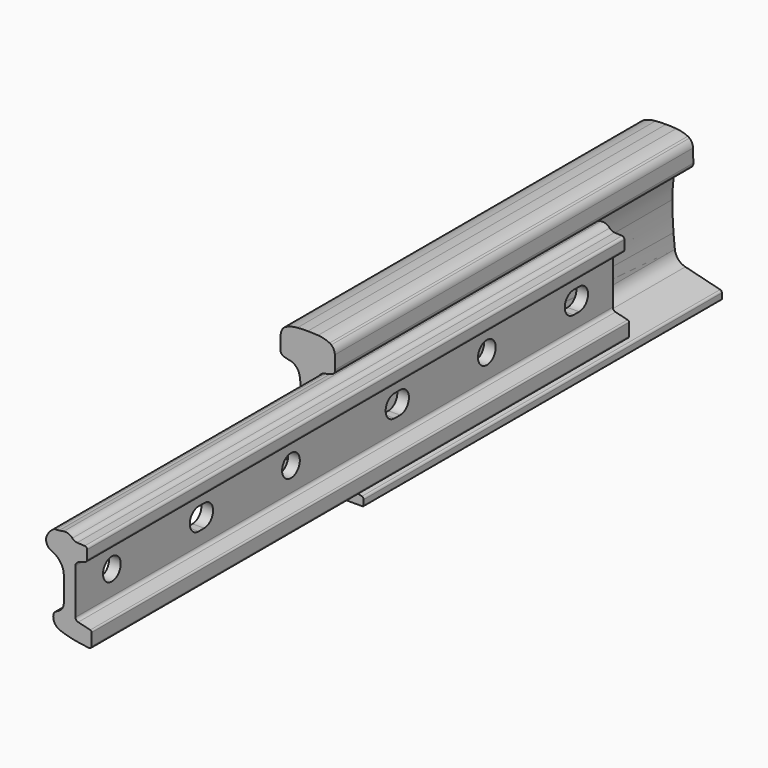
from build123d import *

# Parameters (mm, degrees)
F1_DEPTH  = 609.6
F4_DEPTH  = 609.6
F5_D      = 30.1625
F6_DEPTH  = 609.6
F7_D      = 30.1625
F10_DEPTH = 304.8
F3_R      = 15.08125
F11_DEPTH = 152.401
F12_DEPTH = 457.2
F13_DEPTH = 152.401


with BuildPart() as f1:
    # F0 (on Front) → F1 (new body)
    with BuildSketch(Plane.XZ):
        with BuildLine():
            Line((-74.6125, 0), (0, 0))
            Line((0, 0), (74.6125, 0))
            ThreePointArc((74.6125, 0), (75.7350320151, 0.4649679849), (76.2, 1.5875))
            Line((76.2, 1.5875), (76.2, 8.6375172708))
            ThreePointArc((76.2, 8.6375172708), (75.5275026433, 10.5915145891), (73.7948941606, 11.7177588168))
            Line((73.7948941606, 11.7177588168), (26.4239553104, 23.5579371467))
            ThreePointArc((26.4239553104, 23.5579371467), (16.7305028538, 29.4677613288), (12.1204139211, 39.842544335))
            ThreePointArc((12.1204139211, 39.842544335), (9.5792487577, 69.084794889), (8.73125, 98.425))
            ThreePointArc((8.73125, 98.425), (9.2653580474, 113.148322963), (10.8648744003, 127.7942458741))
            ThreePointArc((10.8648744003, 127.7942458741), (13.5406230824, 135.105519008), (18.917896304, 140.7357302429))
            ThreePointArc((18.917896304, 140.7357302429), (20.1528467839, 141.4316531197), (21.4918904061, 141.8968127872))
            Line((21.4918904061, 141.8968127872), (31.9637779941, 144.5142195666))
            ThreePointArc((31.9637779941, 144.5142195666), (35.8678959033, 147.0868819035), (37.30625, 151.5356868712))
            Line((37.30625, 151.5356868712), (36.8599990785, 169.3703104565))
            ThreePointArc((36.8599990785, 169.3703104565), (35.5405407375, 175.0194624076), (32.0838713197, 179.6783597682))
            ThreePointArc((32.0838713197, 179.6783597682), (30.9805783249, 180.5257181325), (29.765625, 181.2033316273))
            ThreePointArc((29.765625, 181.2033316273), (22.1130671826, 183.945655693), (14.0890625, 185.2484723667))
            ThreePointArc((14.0890625, 185.2484723667), (7.0487734776, 185.6152062911), (0, 185.7375))
            ThreePointArc((0, 185.7375), (-7.0487734776, 185.6152062911), (-14.0890625, 185.2484723667))
            ThreePointArc((-14.0890625, 185.2484723667), (-22.1130671826, 183.945655693), (-29.765625, 181.2033316273))
            ThreePointArc((-29.765625, 181.2033316273), (-30.9805783249, 180.5257181325), (-32.0838713197, 179.6783597682))
            ThreePointArc((-32.0838713197, 179.6783597682), (-35.5405407375, 175.0194624076), (-36.8599990785, 169.3703104565))
            Line((-36.8599990785, 169.3703104565), (-37.30625, 151.5356868712))
            ThreePointArc((-37.30625, 151.5356868712), (-35.8678959033, 147.0868819035), (-31.9637779941, 144.5142195666))
            Line((-31.9637779941, 144.5142195666), (-21.4918904061, 141.8968127872))
            ThreePointArc((-21.4918904061, 141.8968127872), (-20.1528467839, 141.4316531197), (-18.917896304, 140.7357302429))
            ThreePointArc((-18.917896304, 140.7357302429), (-13.5406230824, 135.105519008), (-10.8648744003, 127.7942458741))
            ThreePointArc((-10.8648744003, 127.7942458741), (-9.2653580474, 113.148322963), (-8.73125, 98.425))
            ThreePointArc((-8.73125, 98.425), (-9.5792487577, 69.084794889), (-12.1204139211, 39.842544335))
            ThreePointArc((-12.1204139211, 39.842544335), (-16.7305028538, 29.4677613288), (-26.4239553104, 23.5579371467))
            Line((-26.4239553104, 23.5579371467), (-73.7948941606, 11.7177588168))
            ThreePointArc((-73.7948941606, 11.7177588168), (-75.5275026433, 10.5915145891), (-76.2, 8.6375172708))
            Line((-76.2, 8.6375172708), (-76.2, 1.5875))
            ThreePointArc((-76.2, 1.5875), (-75.7350320151, 0.4649679849), (-74.6125, 0))
        make_face()
    extrude(amount=-F1_DEPTH)


with BuildPart() as f4:
    # F0 (on Front) → F4 (new body)
    with BuildSketch(Plane.XZ):
        with BuildLine():
            Line((-74.6125, 0), (0, 0))
            Line((0, 0), (74.6125, 0))
            ThreePointArc((74.6125, 0), (75.7350320151, 0.4649679849), (76.2, 1.5875))
            Line((76.2, 1.5875), (76.2, 8.6375172708))
            ThreePointArc((76.2, 8.6375172708), (75.5275026433, 10.5915145891), (73.7948941606, 11.7177588168))
            Line((73.7948941606, 11.7177588168), (26.4239553104, 23.5579371467))
            ThreePointArc((26.4239553104, 23.5579371467), (16.7305028538, 29.4677613288), (12.1204139211, 39.842544335))
            ThreePointArc((12.1204139211, 39.842544335), (9.5792487577, 69.084794889), (8.73125, 98.425))
            ThreePointArc((8.73125, 98.425), (9.2653580474, 113.148322963), (10.8648744003, 127.7942458741))
            ThreePointArc((10.8648744003, 127.7942458741), (13.5406230824, 135.105519008), (18.917896304, 140.7357302429))
            ThreePointArc((18.917896304, 140.7357302429), (20.1528467839, 141.4316531197), (21.4918904061, 141.8968127872))
            Line((21.4918904061, 141.8968127872), (31.9637779941, 144.5142195666))
            ThreePointArc((31.9637779941, 144.5142195666), (35.8678959033, 147.0868819035), (37.30625, 151.5356868712))
            Line((37.30625, 151.5356868712), (36.8599990785, 169.3703104565))
            ThreePointArc((36.8599990785, 169.3703104565), (35.5405407375, 175.0194624076), (32.0838713197, 179.6783597682))
            ThreePointArc((32.0838713197, 179.6783597682), (30.9805783249, 180.5257181325), (29.765625, 181.2033316273))
            ThreePointArc((29.765625, 181.2033316273), (22.1130671826, 183.945655693), (14.0890625, 185.2484723667))
            ThreePointArc((14.0890625, 185.2484723667), (7.0487734776, 185.6152062911), (0, 185.7375))
            ThreePointArc((0, 185.7375), (-7.0487734776, 185.6152062911), (-14.0890625, 185.2484723667))
            ThreePointArc((-14.0890625, 185.2484723667), (-22.1130671826, 183.945655693), (-29.765625, 181.2033316273))
            ThreePointArc((-29.765625, 181.2033316273), (-30.9805783249, 180.5257181325), (-32.0838713197, 179.6783597682))
            ThreePointArc((-32.0838713197, 179.6783597682), (-35.5405407375, 175.0194624076), (-36.8599990785, 169.3703104565))
            Line((-36.8599990785, 169.3703104565), (-37.30625, 151.5356868712))
            ThreePointArc((-37.30625, 151.5356868712), (-35.8678959033, 147.0868819035), (-31.9637779941, 144.5142195666))
            Line((-31.9637779941, 144.5142195666), (-21.4918904061, 141.8968127872))
            ThreePointArc((-21.4918904061, 141.8968127872), (-20.1528467839, 141.4316531197), (-18.917896304, 140.7357302429))
            ThreePointArc((-18.917896304, 140.7357302429), (-13.5406230824, 135.105519008), (-10.8648744003, 127.7942458741))
            ThreePointArc((-10.8648744003, 127.7942458741), (-9.2653580474, 113.148322963), (-8.73125, 98.425))
            ThreePointArc((-8.73125, 98.425), (-9.5792487577, 69.084794889), (-12.1204139211, 39.842544335))
            ThreePointArc((-12.1204139211, 39.842544335), (-16.7305028538, 29.4677613288), (-26.4239553104, 23.5579371467))
            Line((-26.4239553104, 23.5579371467), (-73.7948941606, 11.7177588168))
            ThreePointArc((-73.7948941606, 11.7177588168), (-75.5275026433, 10.5915145891), (-76.2, 8.6375172708))
            Line((-76.2, 8.6375172708), (-76.2, 1.5875))
            ThreePointArc((-76.2, 1.5875), (-75.7350320151, 0.4649679849), (-74.6125, 0))
        make_face()
    extrude(amount=-F4_DEPTH)

    # F5 (through all)
    with Locations(Plane.YZ.offset(76.2)):
        with Locations((88.9, 78.58125), (241.3, 78.58125)):
            Hole(F5_D / 2)


with BuildPart() as f6:
    # F0 (on Front) → F6 (new body)
    with BuildSketch(Plane.XZ):
        with BuildLine():
            Line((-74.6125, 0), (0, 0))
            Line((0, 0), (74.6125, 0))
            ThreePointArc((74.6125, 0), (75.7350320151, 0.4649679849), (76.2, 1.5875))
            Line((76.2, 1.5875), (76.2, 8.6375172708))
            ThreePointArc((76.2, 8.6375172708), (75.5275026433, 10.5915145891), (73.7948941606, 11.7177588168))
            Line((73.7948941606, 11.7177588168), (26.4239553104, 23.5579371467))
            ThreePointArc((26.4239553104, 23.5579371467), (16.7305028538, 29.4677613288), (12.1204139211, 39.842544335))
            ThreePointArc((12.1204139211, 39.842544335), (9.5792487577, 69.084794889), (8.73125, 98.425))
            ThreePointArc((8.73125, 98.425), (9.2653580474, 113.148322963), (10.8648744003, 127.7942458741))
            ThreePointArc((10.8648744003, 127.7942458741), (13.5406230824, 135.105519008), (18.917896304, 140.7357302429))
            ThreePointArc((18.917896304, 140.7357302429), (20.1528467839, 141.4316531197), (21.4918904061, 141.8968127872))
            Line((21.4918904061, 141.8968127872), (31.9637779941, 144.5142195666))
            ThreePointArc((31.9637779941, 144.5142195666), (35.8678959033, 147.0868819035), (37.30625, 151.5356868712))
            Line((37.30625, 151.5356868712), (36.8599990785, 169.3703104565))
            ThreePointArc((36.8599990785, 169.3703104565), (35.5405407375, 175.0194624076), (32.0838713197, 179.6783597682))
            ThreePointArc((32.0838713197, 179.6783597682), (30.9805783249, 180.5257181325), (29.765625, 181.2033316273))
            ThreePointArc((29.765625, 181.2033316273), (22.1130671826, 183.945655693), (14.0890625, 185.2484723667))
            ThreePointArc((14.0890625, 185.2484723667), (7.0487734776, 185.6152062911), (0, 185.7375))
            ThreePointArc((0, 185.7375), (-7.0487734776, 185.6152062911), (-14.0890625, 185.2484723667))
            ThreePointArc((-14.0890625, 185.2484723667), (-22.1130671826, 183.945655693), (-29.765625, 181.2033316273))
            ThreePointArc((-29.765625, 181.2033316273), (-30.9805783249, 180.5257181325), (-32.0838713197, 179.6783597682))
            ThreePointArc((-32.0838713197, 179.6783597682), (-35.5405407375, 175.0194624076), (-36.8599990785, 169.3703104565))
            Line((-36.8599990785, 169.3703104565), (-37.30625, 151.5356868712))
            ThreePointArc((-37.30625, 151.5356868712), (-35.8678959033, 147.0868819035), (-31.9637779941, 144.5142195666))
            Line((-31.9637779941, 144.5142195666), (-21.4918904061, 141.8968127872))
            ThreePointArc((-21.4918904061, 141.8968127872), (-20.1528467839, 141.4316531197), (-18.917896304, 140.7357302429))
            ThreePointArc((-18.917896304, 140.7357302429), (-13.5406230824, 135.105519008), (-10.8648744003, 127.7942458741))
            ThreePointArc((-10.8648744003, 127.7942458741), (-9.2653580474, 113.148322963), (-8.73125, 98.425))
            ThreePointArc((-8.73125, 98.425), (-9.5792487577, 69.084794889), (-12.1204139211, 39.842544335))
            ThreePointArc((-12.1204139211, 39.842544335), (-16.7305028538, 29.4677613288), (-26.4239553104, 23.5579371467))
            Line((-26.4239553104, 23.5579371467), (-73.7948941606, 11.7177588168))
            ThreePointArc((-73.7948941606, 11.7177588168), (-75.5275026433, 10.5915145891), (-76.2, 8.6375172708))
            Line((-76.2, 8.6375172708), (-76.2, 1.5875))
            ThreePointArc((-76.2, 1.5875), (-75.7350320151, 0.4649679849), (-74.6125, 0))
        make_face()
    extrude(amount=-F6_DEPTH)

    # F7 (through all)
    with Locations(Plane.YZ.offset(76.2)):
        with Locations((88.9, 78.58125), (241.3, 78.58125), (393.7, 78.58125)):
            Hole(F7_D / 2)


with BuildPart() as f10:
    # F9 (on offset) → F10 (new body, symmetric)
    with BuildSketch(Plane.XZ.offset(1.5875)):
        with BuildLine():
            ThreePointArc((69.0238028765, 14.9720329791), (71.7015465308, 15.7643399473), (72.8598327987, 18.3052914092))
            Line((72.8598327987, 18.3052914092), (72.8598327987, 34.7940649429))
            ThreePointArc((72.8598327987, 34.7940649429), (72.3392500977, 36.2959489919), (71.000849976, 37.1534728456))
            Line((71.000849976, 37.1534728456), (54.4682666659, 41.1319620907))
            ThreePointArc((54.4682666659, 41.1319620907), (51.827247883, 42.8240843252), (50.8, 45.7877003015))
            Line((50.8, 45.7877003015), (50.8, 107.4779679297))
            ThreePointArc((50.8, 107.4779679297), (51.8703010547, 110.8815842809), (54.6959526837, 113.060079515))
            Line((54.6959526837, 113.060079515), (64.3855764499, 116.6203490669))
            ThreePointArc((64.3855764499, 116.6203490669), (66.0200990727, 117.8805184761), (66.6392239744, 119.8493697911))
            Line((66.6392239744, 119.8493697911), (66.6392239744, 131.9592517381))
            ThreePointArc((66.6392239744, 131.9592517381), (65.6910304188, 134.338321302), (63.3663386107, 135.4129612446))
            Line((63.3663386107, 135.4129612446), (53.1041169145, 135.965097777))
            ThreePointArc((53.1041169145, 135.965097777), (49.4922154376, 136.9101924328), (46.5433926041, 139.2000570761))
            ThreePointArc((46.5433926041, 139.2000570761), (41.2194426913, 142.9087406355), (34.7637906671, 143.5593813658))
            Line((34.7637906671, 143.5593813658), (28.5080823248, 142.5911900901))
            ThreePointArc((28.5080823248, 142.5911900901), (26.4769012755, 142.3819095036), (24.4349680387, 142.3800451782))
            ThreePointArc((24.4349680387, 142.3800451782), (21.8792477704, 141.9901504634), (19.6807886431, 140.6298190907))
            ThreePointArc((19.6807886431, 140.6298190907), (19.5778579973, 140.5392485952), (19.4690358738, 140.4558490871))
            ThreePointArc((19.4690358738, 140.4558490871), (16.080406355, 137.477246332), (13.3585447331, 133.8791421505))
            ThreePointArc((13.3585447331, 133.8791421505), (12.4631042599, 132.2727605016), (11.6924308012, 130.6029287546))
            ThreePointArc((11.6924308012, 130.6029287546), (11.727654984, 121.1366917036), (18.5172575143, 114.5403152642))
            ThreePointArc((18.5172575143, 114.5403152642), (30.4320213726, 105.054539508), (34.925, 90.5027464037))
            Line((34.925, 90.5027464037), (34.925, 58.1303172338))
            ThreePointArc((34.925, 58.1303172338), (32.3901124815, 50.0490036177), (25.6937207289, 44.8632903601))
            ThreePointArc((25.6937207289, 44.8632903601), (22.253564155, 42.3656223483), (20.6105513237, 38.4447128126))
            ThreePointArc((20.6105513237, 38.4447128126), (22.5397602678, 29.3741494815), (29.6653751284, 23.4392881393))
            ThreePointArc((29.6653751284, 23.4392881393), (42.180646717, 19.4877347353), (55.0554403421, 16.9408766014))
            Line((55.0554403421, 16.9408766014), (69.0238028765, 14.9720329791))
        make_face()
    extrude(amount=F10_DEPTH, both=True)

    # F3 (on offset) → F11 (cut, through all)
    with BuildSketch(Plane.YZ.offset(76.2)):
        with BuildLine():
            Line((-239.7125, 93.6625), (-249.2375, 93.6625))
            ThreePointArc((-249.2375, 93.6625), (-264.31875, 78.58125), (-249.2375, 63.5))
            Line((-249.2375, 63.5), (-239.7125, 63.5))
            ThreePointArc((-239.7125, 63.5), (-224.63125, 78.58125), (-239.7125, 93.6625))
        make_face()
        with Locations((-92.075, 78.58125)):
            Circle(F3_R)
        with BuildLine():
            Line((93.6625, 93.6625), (84.1375, 93.6625))
            ThreePointArc((84.1375, 93.6625), (69.05625, 78.58125), (84.1375, 63.5))
            Line((84.1375, 63.5), (93.6625, 63.5))
            ThreePointArc((93.6625, 63.5), (108.74375, 78.58125), (93.6625, 93.6625))
        make_face()
        with Locations((241.3, 78.58125)):
            Circle(F3_R)
    extrude(amount=-F11_DEPTH, mode=Mode.SUBTRACT)


with BuildPart() as f12:
    # F9 (on offset) → F12 (new body, symmetric)
    with BuildSketch(Plane.XZ.offset(1.5875)):
        with BuildLine():
            ThreePointArc((69.0238028765, 14.9720329791), (71.7015465308, 15.7643399473), (72.8598327987, 18.3052914092))
            Line((72.8598327987, 18.3052914092), (72.8598327987, 34.7940649429))
            ThreePointArc((72.8598327987, 34.7940649429), (72.3392500977, 36.2959489919), (71.000849976, 37.1534728456))
            Line((71.000849976, 37.1534728456), (54.4682666659, 41.1319620907))
            ThreePointArc((54.4682666659, 41.1319620907), (51.827247883, 42.8240843252), (50.8, 45.7877003015))
            Line((50.8, 45.7877003015), (50.8, 107.4779679297))
            ThreePointArc((50.8, 107.4779679297), (51.8703010547, 110.8815842809), (54.6959526837, 113.060079515))
            Line((54.6959526837, 113.060079515), (64.3855764499, 116.6203490669))
            ThreePointArc((64.3855764499, 116.6203490669), (66.0200990727, 117.8805184761), (66.6392239744, 119.8493697911))
            Line((66.6392239744, 119.8493697911), (66.6392239744, 131.9592517381))
            ThreePointArc((66.6392239744, 131.9592517381), (65.6910304188, 134.338321302), (63.3663386107, 135.4129612446))
            Line((63.3663386107, 135.4129612446), (53.1041169145, 135.965097777))
            ThreePointArc((53.1041169145, 135.965097777), (49.4922154376, 136.9101924328), (46.5433926041, 139.2000570761))
            ThreePointArc((46.5433926041, 139.2000570761), (41.2194426913, 142.9087406355), (34.7637906671, 143.5593813658))
            Line((34.7637906671, 143.5593813658), (28.5080823248, 142.5911900901))
            ThreePointArc((28.5080823248, 142.5911900901), (26.4769012755, 142.3819095036), (24.4349680387, 142.3800451782))
            ThreePointArc((24.4349680387, 142.3800451782), (21.8792477704, 141.9901504634), (19.6807886431, 140.6298190907))
            ThreePointArc((19.6807886431, 140.6298190907), (19.5778579973, 140.5392485952), (19.4690358738, 140.4558490871))
            ThreePointArc((19.4690358738, 140.4558490871), (16.080406355, 137.477246332), (13.3585447331, 133.8791421505))
            ThreePointArc((13.3585447331, 133.8791421505), (12.4631042599, 132.2727605016), (11.6924308012, 130.6029287546))
            ThreePointArc((11.6924308012, 130.6029287546), (11.727654984, 121.1366917036), (18.5172575143, 114.5403152642))
            ThreePointArc((18.5172575143, 114.5403152642), (30.4320213726, 105.054539508), (34.925, 90.5027464037))
            Line((34.925, 90.5027464037), (34.925, 58.1303172338))
            ThreePointArc((34.925, 58.1303172338), (32.3901124815, 50.0490036177), (25.6937207289, 44.8632903601))
            ThreePointArc((25.6937207289, 44.8632903601), (22.253564155, 42.3656223483), (20.6105513237, 38.4447128126))
            ThreePointArc((20.6105513237, 38.4447128126), (22.5397602678, 29.3741494815), (29.6653751284, 23.4392881393))
            ThreePointArc((29.6653751284, 23.4392881393), (42.180646717, 19.4877347353), (55.0554403421, 16.9408766014))
            Line((55.0554403421, 16.9408766014), (69.0238028765, 14.9720329791))
        make_face()
    extrude(amount=F12_DEPTH, both=True)

    # F3 (on offset) → F13 (cut, through all)
    with BuildSketch(Plane.YZ.offset(76.2)):
        with Locations((-396.875, 78.58125)):
            Circle(F3_R)
        with BuildLine():
            Line((-239.7125, 93.6625), (-249.2375, 93.6625))
            ThreePointArc((-249.2375, 93.6625), (-264.31875, 78.58125), (-249.2375, 63.5))
            Line((-249.2375, 63.5), (-239.7125, 63.5))
            ThreePointArc((-239.7125, 63.5), (-224.63125, 78.58125), (-239.7125, 93.6625))
        make_face()
        with Locations((-92.075, 78.58125)):
            Circle(F3_R)
        with BuildLine():
            Line((93.6625, 93.6625), (84.1375, 93.6625))
            ThreePointArc((84.1375, 93.6625), (69.05625, 78.58125), (84.1375, 63.5))
            Line((84.1375, 63.5), (93.6625, 63.5))
            ThreePointArc((93.6625, 63.5), (108.74375, 78.58125), (93.6625, 93.6625))
        make_face()
        with Locations((241.3, 78.58125)):
            Circle(F3_R)
        with BuildLine():
            Line((398.4625, 93.6625), (388.9375, 93.6625))
            ThreePointArc((388.9375, 93.6625), (373.85625, 78.58125), (388.9375, 63.5))
            Line((388.9375, 63.5), (398.4625, 63.5))
            ThreePointArc((398.4625, 63.5), (413.54375, 78.58125), (398.4625, 93.6625))
        make_face()
    extrude(amount=-F13_DEPTH, mode=Mode.SUBTRACT)


solid = Compound([f1.part, f4.part, f6.part, f10.part, f12.part])
